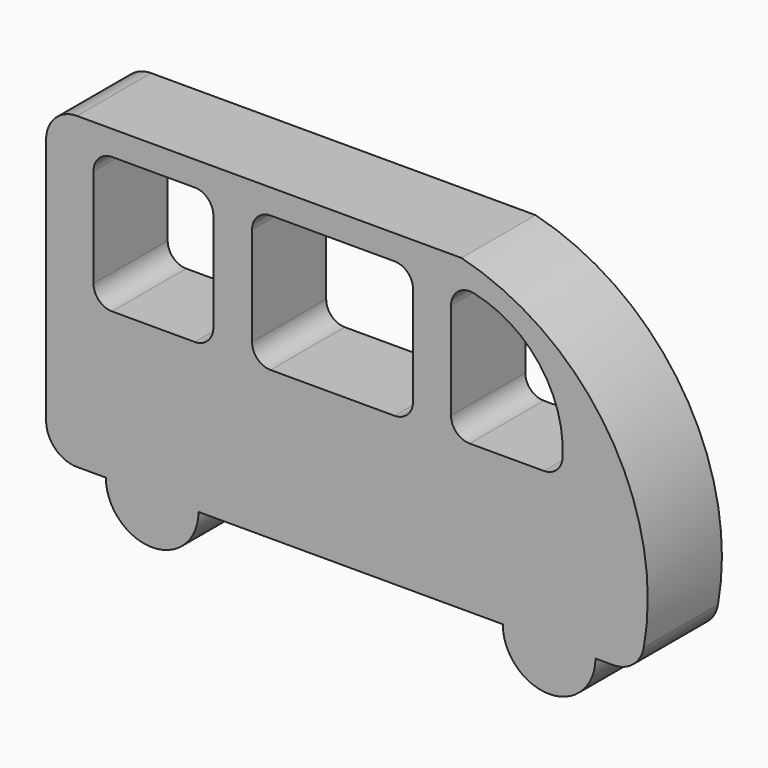
from build123d import *

# Parameters (mm, degrees)
F1_DEPTH = 15


# Not quite as in the source:
# - a feature names something its author has since deleted; it is built from what else it names


with BuildPart() as f1:
    # F0 (on Front) → F1 (new body)
    with BuildSketch(Plane.XZ):
        with BuildLine():
            Line((45.2788062093, 66.612446636), (-16.9345241785, 66.612446636))
            ThreePointArc((-16.9345241785, 66.612446636), (-20.4700580844, 65.1479805419), (-21.9345241785, 61.612446636))
            Line((-21.9345241785, 61.612446636), (-21.9345241785, 21.612446636))
            ThreePointArc((-21.9345241785, 21.612446636), (-20.4700580844, 18.07691273), (-16.9345241785, 16.612446636))
            Line((-16.9345241785, 16.612446636), (-12.2681620345, 16.612446636))
            ThreePointArc((-12.2681620345, 16.612446636), (-4.7681620345, 9.112446636), (2.7318379655, 16.612446636))
            Line((2.7318379655, 16.612446636), (51.954228729, 16.612446636))
            ThreePointArc((51.954228729, 16.612446636), (59.454228729, 9.112446636), (66.954228729, 16.612446636))
            Line((66.954228729, 16.612446636), (69.8528067806, 16.612446636))
            ThreePointArc((69.8528067806, 16.612446636), (73.0579467169, 17.774859114), (74.7728087909, 20.7216154405))
            ThreePointArc((74.7728087909, 20.7216154405), (69.0623483383, 49.4748090163), (45.2788062093, 66.612446636))
        make_face()
        with BuildLine():
            ThreePointArc((-14.2601495609, 59.612446636), (-13.3814699044, 61.7337669795), (-11.2601495609, 62.612446636))
            Line((-11.2601495609, 62.612446636), (2.1277400926, 62.612446636))
            ThreePointArc((2.1277400926, 62.612446636), (4.2490604361, 61.7337669795), (5.1277400926, 59.612446636))
            Line((5.1277400926, 59.612446636), (5.1277400926, 43.612446636))
            ThreePointArc((5.1277400926, 43.612446636), (4.2490604361, 41.4911262924), (2.1277400926, 40.612446636))
            Line((2.1277400926, 40.612446636), (-11.2601495609, 40.612446636))
            ThreePointArc((-11.2601495609, 40.612446636), (-13.3814699044, 41.4911262924), (-14.2601495609, 43.612446636))
            Line((-14.2601495609, 43.612446636), (-14.2601495609, 59.612446636))
        make_face(mode=Mode.SUBTRACT)
        with BuildLine():
            ThreePointArc((11.388416402, 59.612446636), (12.2670960585, 61.7337669795), (14.388416402, 62.612446636))
            Line((14.388416402, 62.612446636), (34.4408885837, 62.612446636))
            ThreePointArc((34.4408885837, 62.612446636), (36.5622089272, 61.7337669795), (37.4408885837, 59.612446636))
            Line((37.4408885837, 59.612446636), (37.4408885837, 43.612446636))
            ThreePointArc((37.4408885837, 43.612446636), (36.5622089272, 41.4911262924), (34.4408885837, 40.612446636))
            Line((34.4408885837, 40.612446636), (14.388416402, 40.612446636))
            ThreePointArc((14.388416402, 40.612446636), (12.2670960585, 41.4911262924), (11.388416402, 43.612446636))
            Line((11.388416402, 43.612446636), (11.388416402, 59.612446636))
        make_face(mode=Mode.SUBTRACT)
        with BuildLine():
            ThreePointArc((61.6208599434, 43.4263003167), (60.6810944136, 41.4263040334), (58.626640588, 40.612446636))
            Line((58.626640588, 40.612446636), (46.5931359261, 40.612446636))
            ThreePointArc((46.5931359261, 40.612446636), (44.4718155826, 41.4911262924), (43.5931359261, 43.612446636))
            Line((43.5931359261, 43.612446636), (43.5931359261, 59.3101777172))
            ThreePointArc((43.5931359261, 59.3101777172), (44.6949543188, 61.6333020328), (47.1910736498, 62.2499856155))
            ThreePointArc((47.1910736498, 62.2499856155), (57.9277499616, 55.5378575882), (61.6208599434, 43.4263003167))
        make_face(mode=Mode.SUBTRACT)
    extrude(amount=F1_DEPTH)


solid = f1.part
